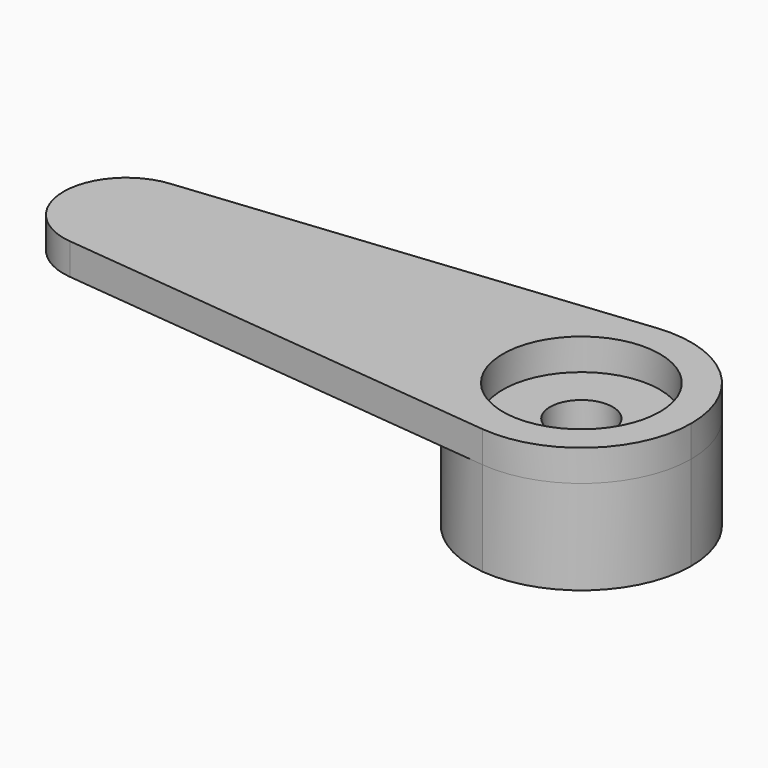
from build123d import *
from build123d import SkipClean  # not in build123d's __all__

# Parameters (mm, degrees)
F0_R     = 2.5
F1_DEPTH = 1
F2_DEPTH = 3
F0_R_2   = 1
F3_DEPTH = 1


# Not quite as in the source:
# - after a boolean that leaves OpenCascade's solid faulty, fix() repairs it


with BuildPart() as f1:
    # F0 (on Top) → F1 (new body)
    with BuildSketch(Plane.XY):
        with BuildLine():
            ThreePointArc((-12.5, 0), (-13.1609318732, 1.4855627054), (-14.7068965517, 1.9892696692))
            ThreePointArc((-14.7068965517, 1.9892696692), (-16.5, 0), (-14.7068965517, -1.9892696692))
            ThreePointArc((-14.7068965517, -1.9892696692), (-13.1609318732, -1.4855627054), (-12.5, 0))
        make_face()
        with BuildLine():
            ThreePointArc((-0.362068922, -3.4812219257), (-3.5, 7.5e-09), (-0.362068907, 3.4812219272))
            Line((-0.362068907, 3.4812219272), (-14.7068965517, 1.9892696692))
            ThreePointArc((-14.7068965517, 1.9892696692), (-13.1609318732, 1.4855627054), (-12.5, 0))
            ThreePointArc((-12.5, 0), (-13.1609318732, -1.4855627054), (-14.7068965517, -1.9892696692))
            Line((-14.7068965517, -1.9892696692), (-0.362068922, -3.4812219257))
        make_face()
        with BuildLine():
            ThreePointArc((-0.362068922, -3.4812219257), (2.3433692382, -2.5997347198), (3.5, 0))
            ThreePointArc((3.5, 0), (2.3433692438, 2.5997347148), (-0.362068907, 3.4812219272))
            ThreePointArc((-0.362068907, 3.4812219272), (-3.5, 7.5e-09), (-0.362068922, -3.4812219257))
        make_face()
        Circle(F0_R, mode=Mode.SUBTRACT)
    extrude(amount=F1_DEPTH)

    # F0 (on Top) → F2 (join)
    with BuildSketch(Plane.XY):
        with BuildLine():
            ThreePointArc((-0.362068922, -3.4812219257), (2.3433692382, -2.5997347198), (3.5, 0))
            ThreePointArc((3.5, 0), (2.3433692438, 2.5997347148), (-0.362068907, 3.4812219272))
            ThreePointArc((-0.362068907, 3.4812219272), (-3.5, 7.5e-09), (-0.362068922, -3.4812219257))
        make_face()
        Circle(F0_R, mode=Mode.SUBTRACT)
    with SkipClean():  # cleaning this boolean's faces spoils the solid; the shape is the same uncleaned
        extrude(amount=-F2_DEPTH)

    # F0 (on Top) → F3 (join)
    with BuildSketch(Plane.XY):
        Circle(F0_R)
        Circle(F0_R_2, mode=Mode.SUBTRACT)
    extrude(amount=-F3_DEPTH)

    add(f1.part.fix(), mode=Mode.REPLACE)


solid = f1.part
